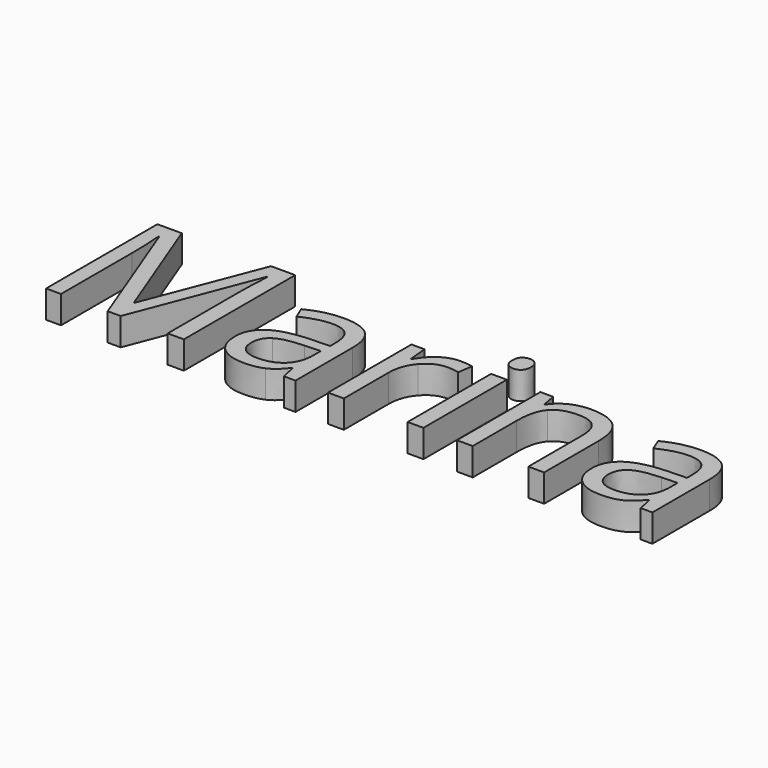
from build123d import *

# Parameters (mm, degrees)
F0_W     = 2.9069138788
F0_H     = 19.1833912039
F1_DEPTH = 5.08


with BuildPart() as f1:
    # F0 (on Top) → F1 (new body)
    with BuildSketch(Plane.XY):
        with BuildLine():
            add(Edge.make_bspline(
                [(-10.535576719, -11.46055758), (-10.5188298141, -11.4434207138), (-10.5014678379, -11.4269516392)],
                knots=[0.9645736592, 0.9645736592, 0.9645736592, 1, 1, 1], degree=2))
            Line((-10.535576719, -11.46055758), (-8.0387668081, -11.46055758))
            add(Edge.make_bspline(
                [(-8.0650371302, -11.4353531244), (-8.0517272234, -11.4477806064), (-8.0387668081, -11.46055758)],
                knots=[0, 0, 0, 0.026257999, 0.026257999, 0.026257999], degree=2))
            add(Edge.make_bspline(
                [(-9.2720505038, -10.9620694582), (-8.5719267372, -10.9620694582), (-8.0650371302, -11.4353531244)],
                knots=[0, 0, 0, 1, 1, 1], degree=2))
            add(Edge.make_bspline(
                [(-10.5014678379, -11.4269516392), (-10.0113812013, -10.9620694582), (-9.2720505038, -10.9620694582)],
                knots=[0, 0, 0, 1, 1, 1], degree=2))
        make_face()
        with BuildLine():
            Line((-8.0387668081, -11.46055758), (-10.535576719, -11.46055758))
            add(Edge.make_bspline(
                [(-10.9915544745, -12.8888100638), (-10.9915544745, -11.9271530403), (-10.535576719, -11.46055758)],
                knots=[0, 0, 0, 0.9645736592, 0.9645736592, 0.9645736592], degree=2))
            add(Edge.make_bspline(
                [(-10.5014678379, -14.3506684884), (-10.9915544745, -13.868983337), (-10.9915544745, -12.8888100638)],
                knots=[0, 0, 0, 1, 1, 1], degree=2))
            add(Edge.make_bspline(
                [(-9.2720505038, -14.8323536398), (-10.0113812013, -14.8323536398), (-10.5014678379, -14.3506684884)],
                knots=[0, 0, 0, 1, 1, 1], degree=2))
            add(Edge.make_bspline(
                [(-8.0650371302, -14.3506684884), (-8.5719267372, -14.8323536398), (-9.2720505038, -14.8323536398)],
                knots=[0, 0, 0, 1, 1, 1], degree=2))
            add(Edge.make_bspline(
                [(-7.5581475232, -12.8888100638), (-7.5581475232, -13.868983337), (-8.0650371302, -14.3506684884)],
                knots=[0, 0, 0, 1, 1, 1], degree=2))
            add(Edge.make_bspline(
                [(-8.0387668081, -11.46055758), (-7.5581475232, -11.9343741794), (-7.5581475232, -12.8888100638)],
                knots=[0.026257999, 0.026257999, 0.026257999, 1, 1, 1], degree=2))
        make_face()
        with BuildLine():
            Line((-74.5963984195, -14.5859100739), (-65.9148637141, -37.2699201107))
            Line((-65.9148637141, -37.2699201107), (-63.5176399373, -37.2699201107))
            Line((-63.5176399373, -37.2699201107), (-54.7632923602, -14.6195160147))
            Line((-54.7632923602, -14.6195160147), (-54.6232676069, -14.6195160147))
            add(Edge.make_bspline(
                [(-54.8697111727, -20.7806051605), (-54.8697111727, -17.9465041535), (-54.6232676069, -14.6195160147)],
                knots=[0, 0, 0, 1, 1, 1], degree=2))
            Line((-54.8697111727, -20.7806051605), (-54.8697111727, -37.2699201107))
            Line((-54.8697111727, -37.2699201107), (-51.8955854123, -37.2699201107))
            Line((-51.8955854123, -37.2699201107), (-51.8955854123, -11.6789961952))
            Line((-51.8955854123, -11.6789961952), (-56.3427715776, -11.6789961952))
            Line((-56.3427715776, -11.6789961952), (-64.5146161809, -32.7891280047))
            Line((-64.5146161809, -32.7891280047), (-64.6546409342, -32.7891280047))
            Line((-64.6546409342, -32.7891280047), (-72.759273656, -11.6789961952))
            Line((-72.759273656, -11.6789961952), (-77.240065762, -11.6789961952))
            Line((-77.240065762, -11.6789961952), (-77.240065762, -37.2699201107))
            Line((-77.240065762, -37.2699201107), (-74.489979607, -37.2699201107))
            Line((-74.489979607, -37.2699201107), (-74.489979607, -20.9934427856))
            add(Edge.make_bspline(
                [(-74.7364231728, -14.5859100739), (-74.489979607, -17.2799863277), (-74.489979607, -20.9934427856)],
                knots=[0, 0, 0, 1, 1, 1], degree=2))
            Line((-74.7364231728, -14.5859100739), (-74.5963984195, -14.5859100739))
        make_face()
        with BuildLine():
            Line((-34.0956387712, -34.536636926), (-33.5187367875, -37.2699201107))
            Line((-33.5187367875, -37.2699201107), (-31.3623555865, -37.2699201107))
            Line((-31.3623555865, -37.2699201107), (-31.3623555865, -24.1748051808))
            add(Edge.make_bspline(
                [(-33.0174481706, -19.2935422803), (-31.3623555865, -20.8142111013), (-31.3623555865, -24.1748051808)],
                knots=[0, 0, 0, 1, 1, 1], degree=2))
            add(Edge.make_bspline(
                [(-38.1003467159, -17.7728734594), (-34.6725407548, -17.7728734594), (-33.0174481706, -19.2935422803)],
                knots=[0, 0, 0, 1, 1, 1], degree=2))
            add(Edge.make_bspline(
                [(-41.4917462412, -18.2097506897), (-39.8030477162, -17.7728734594), (-38.1003467159, -17.7728734594)],
                knots=[0, 0, 0, 1, 1, 1], degree=2))
            add(Edge.make_bspline(
                [(-44.5974952697, -19.4139635682), (-43.1804447661, -18.64662792), (-41.4917462412, -18.2097506897)],
                knots=[0, 0, 0, 1, 1, 1], degree=2))
            Line((-44.5974952697, -19.4139635682), (-43.7013368484, -21.6375566508))
            add(Edge.make_bspline(
                [(-38.2795784002, -20.1700972361), (-40.6768021769, -20.1700972361), (-43.7013368484, -21.6375566508)],
                knots=[0, 0, 0, 1, 1, 1], degree=2))
            add(Edge.make_bspline(
                [(-35.1710288766, -21.2454873415), (-36.1400001695, -20.1700972361), (-38.2795784002, -20.1700972361)],
                knots=[0, 0, 0, 1, 1, 1], degree=2))
            add(Edge.make_bspline(
                [(-34.2020575837, -24.5780764704), (-34.2020575837, -22.320877447), (-35.1710288766, -21.2454873415)],
                knots=[0, 0, 0, 1, 1, 1], degree=2))
            Line((-34.2020575837, -24.5780764704), (-34.2020575837, -25.7710873686))
            Line((-34.2020575837, -25.7710873686), (-37.4562328507, -25.8775061811))
            add(Edge.make_bspline(
                [(-46.7482754805, -31.9657824552), (-46.7482754805, -26.1575556878), (-37.4562328507, -25.8775061811)],
                knots=[0, 0, 0, 1, 1, 1], degree=2))
            add(Edge.make_bspline(
                [(-45.1295893322, -36.1497220842), (-46.7482754805, -34.6766616793), (-46.7482754805, -31.9657824552)],
                knots=[0, 0, 0, 1, 1, 1], degree=2))
            add(Edge.make_bspline(
                [(-40.6599992065, -37.6227824891), (-43.5109031839, -37.6227824891), (-45.1295893322, -36.1497220842)],
                knots=[0, 0, 0, 1, 1, 1], degree=2))
            add(Edge.make_bspline(
                [(-37.0949689871, -36.9814691189), (-38.5204209759, -37.6227824891), (-40.6599992065, -37.6227824891)],
                knots=[0, 0, 0, 1, 1, 1], degree=2))
            add(Edge.make_bspline(
                [(-34.2356635245, -34.536636926), (-35.6695169984, -36.3401557487), (-37.0949689871, -36.9814691189)],
                knots=[0, 0, 0, 1, 1, 1], degree=2))
            Line((-34.2356635245, -34.536636926), (-34.0956387712, -34.536636926))
        make_face()
        with BuildLine():
            add(Edge.make_bspline(
                [(-40.0830972228, -35.2199577222), (-37.3666170086, -35.2199577222), (-35.8179432369, -33.732894842)],
                knots=[0, 0, 0, 1, 1, 1], degree=2))
            add(Edge.make_bspline(
                [(-42.7491685259, -34.3994126678), (-41.7970002034, -35.2199577222), (-40.0830972228, -35.2199577222)],
                knots=[0, 0, 0, 1, 1, 1], degree=2))
            add(Edge.make_bspline(
                [(-43.7013368484, -31.999388396), (-43.7013368484, -33.5788676134), (-42.7491685259, -34.3994126678)],
                knots=[0, 0, 0, 1, 1, 1], degree=2))
            add(Edge.make_bspline(
                [(-42.1722665423, -29.0336641208), (-43.7013368484, -29.9886329384), (-43.7013368484, -31.999388396)],
                knots=[0, 0, 0, 1, 1, 1], degree=2))
            add(Edge.make_bspline(
                [(-37.176183344, -27.9554735203), (-40.6431962361, -28.0786953032), (-42.1722665423, -29.0336641208)],
                knots=[0, 0, 0, 1, 1, 1], degree=2))
            Line((-37.176183344, -27.9554735203), (-34.2692694653, -27.8378527275))
            Line((-34.2692694653, -27.8378527275), (-34.2692694653, -29.5685586785))
            add(Edge.make_bspline(
                [(-35.8179432369, -33.732894842), (-34.2692694653, -32.2458319618), (-34.2692694653, -29.5685586785)],
                knots=[0, 0, 0, 1, 1, 1], degree=2))
        make_face(mode=Mode.SUBTRACT)
        with BuildLine():
            add(Edge.make_bspline(
                [(-16.6261505478, -17.7336665284), (-15.3491247976, -17.7336665284), (-14.3353455836, -17.9465041535)],
                knots=[0, 0, 0, 1, 1, 1], degree=2))
            add(Edge.make_bspline(
                [(-19.9363357161, -18.7502462375), (-18.4296693705, -17.7336665284), (-16.6261505478, -17.7336665284)],
                knots=[0, 0, 0, 1, 1, 1], degree=2))
            add(Edge.make_bspline(
                [(-22.5071901869, -21.6375566508), (-21.4430020618, -19.7668259465), (-19.9363357161, -18.7502462375)],
                knots=[0, 0, 0, 1, 1, 1], degree=2))
            Line((-22.5071901869, -21.6375566508), (-22.6472149403, -21.6375566508))
            Line((-22.6472149403, -21.6375566508), (-22.9832743482, -18.0865289068))
            Line((-22.9832743482, -18.0865289068), (-25.3804981249, -18.0865289068))
            Line((-25.3804981249, -18.0865289068), (-25.3804981249, -37.2699201107))
            Line((-25.3804981249, -37.2699201107), (-22.4735842461, -37.2699201107))
            Line((-22.4735842461, -37.2699201107), (-22.4735842461, -26.9753002471))
            add(Edge.make_bspline(
                [(-20.8212921571, -22.2676680407), (-22.4735842461, -24.1580022104), (-22.4735842461, -26.9753002471)],
                knots=[0, 0, 0, 1, 1, 1], degree=2))
            add(Edge.make_bspline(
                [(-16.8389881728, -20.377333871), (-19.169000068, -20.377333871), (-20.8212921571, -22.2676680407)],
                knots=[0, 0, 0, 1, 1, 1], degree=2))
            add(Edge.make_bspline(
                [(-14.7386168731, -20.6405804072), (-15.9260267812, -20.377333871), (-16.8389881728, -20.377333871)],
                knots=[0, 0, 0, 1, 1, 1], degree=2))
            Line((-14.7386168731, -20.6405804072), (-14.3353455836, -17.9465041535))
        make_face()
        with Locations((-9.2916539692, -27.6782245087)):
            Rectangle(F0_W, F0_H)
        with BuildLine():
            Line((11.4516129866, -24.858125977), (11.4516129866, -37.2699201107))
            Line((11.4516129866, -37.2699201107), (14.3585268654, -37.2699201107))
            Line((14.3585268654, -37.2699201107), (14.3585268654, -24.7573081546))
            add(Edge.make_bspline(
                [(12.608217449, -19.405562083), (14.3585268654, -21.0774576376), (14.3585268654, -24.7573081546)],
                knots=[0, 0, 0, 1, 1, 1], degree=2))
            add(Edge.make_bspline(
                [(7.3908951405, -17.7336665284), (10.8579080325, -17.7336665284), (12.608217449, -19.405562083)],
                knots=[0, 0, 0, 1, 1, 1], degree=2))
            add(Edge.make_bspline(
                [(3.8034609606, -18.5150046519), (5.4137456237, -17.7336665284), (7.3908951405, -17.7336665284)],
                knots=[0, 0, 0, 1, 1, 1], degree=2))
            add(Edge.make_bspline(
                [(1.2970178763, -20.7133932789), (2.1931762975, -19.2963427754), (3.8034609606, -18.5150046519)],
                knots=[0, 0, 0, 1, 1, 1], degree=2))
            Line((1.2970178763, -20.7133932789), (1.156993123, -20.7133932789))
            Line((1.156993123, -20.7133932789), (0.6865099519, -18.0865289068))
            Line((0.6865099519, -18.0865289068), (-1.6771078841, -18.0865289068))
            Line((-1.6771078841, -18.0865289068), (-1.6771078841, -37.2699201107))
            Line((-1.6771078841, -37.2699201107), (1.2298059947, -37.2699201107))
            Line((1.2298059947, -37.2699201107), (1.2298059947, -27.2049408425))
            add(Edge.make_bspline(
                [(2.6300535279, -21.8307908104), (1.2298059947, -23.4578784439), (1.2298059947, -27.2049408425)],
                knots=[0, 0, 0, 1, 1, 1], degree=2))
            add(Edge.make_bspline(
                [(7.0380327622, -20.2037031769), (4.030301061, -20.2037031769), (2.6300535279, -21.8307908104)],
                knots=[0, 0, 0, 1, 1, 1], degree=2))
            add(Edge.make_bspline(
                [(10.3846243664, -21.3603076392), (9.3176357461, -20.2037031769), (7.0380327622, -20.2037031769)],
                knots=[0, 0, 0, 1, 1, 1], degree=2))
            add(Edge.make_bspline(
                [(11.4516129866, -24.858125977), (11.4516129866, -22.5169121016), (10.3846243664, -21.3603076392)],
                knots=[0, 0, 0, 1, 1, 1], degree=2))
        make_face()
        with BuildLine():
            Line((31.542364592, -34.536636926), (32.1192665756, -37.2699201107))
            Line((32.1192665756, -37.2699201107), (34.2756477767, -37.2699201107))
            Line((34.2756477767, -37.2699201107), (34.2756477767, -24.1748051808))
            add(Edge.make_bspline(
                [(32.6205551925, -19.2935422803), (34.2756477767, -20.8142111013), (34.2756477767, -24.1748051808)],
                knots=[0, 0, 0, 1, 1, 1], degree=2))
            add(Edge.make_bspline(
                [(27.5376566472, -17.7728734594), (30.9654626083, -17.7728734594), (32.6205551925, -19.2935422803)],
                knots=[0, 0, 0, 1, 1, 1], degree=2))
            add(Edge.make_bspline(
                [(24.146257122, -18.2097506897), (25.8349556469, -17.7728734594), (27.5376566472, -17.7728734594)],
                knots=[0, 0, 0, 1, 1, 1], degree=2))
            add(Edge.make_bspline(
                [(21.0405080935, -19.4139635682), (22.457558597, -18.64662792), (24.146257122, -18.2097506897)],
                knots=[0, 0, 0, 1, 1, 1], degree=2))
            Line((21.0405080935, -19.4139635682), (21.9366665147, -21.6375566508))
            add(Edge.make_bspline(
                [(27.358424963, -20.1700972361), (24.9612011863, -20.1700972361), (21.9366665147, -21.6375566508)],
                knots=[0, 0, 0, 1, 1, 1], degree=2))
            add(Edge.make_bspline(
                [(30.4669744865, -21.2454873415), (29.4980031936, -20.1700972361), (27.358424963, -20.1700972361)],
                knots=[0, 0, 0, 1, 1, 1], degree=2))
            add(Edge.make_bspline(
                [(31.4359457795, -24.5780764704), (31.4359457795, -22.320877447), (30.4669744865, -21.2454873415)],
                knots=[0, 0, 0, 1, 1, 1], degree=2))
            Line((31.4359457795, -24.5780764704), (31.4359457795, -25.7710873686))
            Line((31.4359457795, -25.7710873686), (28.1817705125, -25.8775061811))
            add(Edge.make_bspline(
                [(18.8897278826, -31.9657824552), (18.8897278826, -26.1575556878), (28.1817705125, -25.8775061811)],
                knots=[0, 0, 0, 1, 1, 1], degree=2))
            add(Edge.make_bspline(
                [(20.5084140309, -36.1497220842), (18.8897278826, -34.6766616793), (18.8897278826, -31.9657824552)],
                knots=[0, 0, 0, 1, 1, 1], degree=2))
            add(Edge.make_bspline(
                [(24.9780041567, -37.6227824891), (22.1271001792, -37.6227824891), (20.5084140309, -36.1497220842)],
                knots=[0, 0, 0, 1, 1, 1], degree=2))
            add(Edge.make_bspline(
                [(28.543034376, -36.9814691189), (27.1175823873, -37.6227824891), (24.9780041567, -37.6227824891)],
                knots=[0, 0, 0, 1, 1, 1], degree=2))
            add(Edge.make_bspline(
                [(31.4023398387, -34.536636926), (29.9684863647, -36.3401557487), (28.543034376, -36.9814691189)],
                knots=[0, 0, 0, 1, 1, 1], degree=2))
            Line((31.4023398387, -34.536636926), (31.542364592, -34.536636926))
        make_face()
        with BuildLine():
            add(Edge.make_bspline(
                [(25.5549061403, -35.2199577222), (28.2713863546, -35.2199577222), (29.8200601262, -33.732894842)],
                knots=[0, 0, 0, 1, 1, 1], degree=2))
            add(Edge.make_bspline(
                [(22.8888348372, -34.3994126678), (23.8410031598, -35.2199577222), (25.5549061403, -35.2199577222)],
                knots=[0, 0, 0, 1, 1, 1], degree=2))
            add(Edge.make_bspline(
                [(21.9366665147, -31.999388396), (21.9366665147, -33.5788676134), (22.8888348372, -34.3994126678)],
                knots=[0, 0, 0, 1, 1, 1], degree=2))
            add(Edge.make_bspline(
                [(23.4657368209, -29.0336641208), (21.9366665147, -29.9886329384), (21.9366665147, -31.999388396)],
                knots=[0, 0, 0, 1, 1, 1], degree=2))
            add(Edge.make_bspline(
                [(28.4618200191, -27.9554735203), (24.9948071271, -28.0786953032), (23.4657368209, -29.0336641208)],
                knots=[0, 0, 0, 1, 1, 1], degree=2))
            Line((28.4618200191, -27.9554735203), (31.3687338979, -27.8378527275))
            Line((31.3687338979, -27.8378527275), (31.3687338979, -29.5685586785))
            add(Edge.make_bspline(
                [(29.8200601262, -33.732894842), (31.3687338979, -32.2458319618), (31.3687338979, -29.5685586785)],
                knots=[0, 0, 0, 1, 1, 1], degree=2))
        make_face(mode=Mode.SUBTRACT)
    extrude(amount=F1_DEPTH)


solid = f1.part
